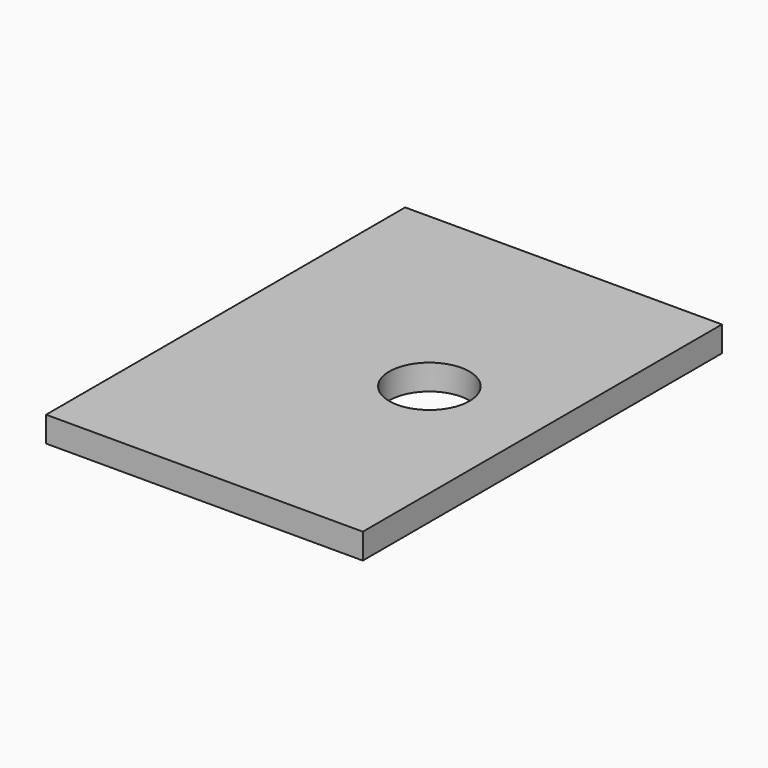
from build123d import *

# Parameters (mm, degrees)
F0_R     = 10
F1_DEPTH = 6.35
F2_W     = 124.221875
F2_H     = 111.91875
F2_R     = 10
F3_DEPTH = 6.351


# Not quite as in the source:
# - a feature names something its author has since deleted; it is built from what else it names


with BuildPart() as f1:
    # F0 (on Top) → F1 (new body)
    with BuildSketch(Plane.XY):
        Polygon((50.8, -55.959375), (50.8, 55.959375), (-50.8, 55.959375), (-152.4, 55.959375), (-152.4, -55.959375), (-50.8, -55.959375), align=None)
        with Locations((-101.6, 0)):
            Circle(F0_R, mode=Mode.SUBTRACT)
        Circle(F0_R, mode=Mode.SUBTRACT)
    extrude(amount=F1_DEPTH)

    # F2 (on face) → F3 (cut, through all)
    with BuildSketch(Plane.XY.offset(6.35)):
        with Locations((-11.3109375, 0)):
            Rectangle(F2_W, F2_H)
        Circle(F2_R, mode=Mode.SUBTRACT)
    extrude(amount=-F3_DEPTH, mode=Mode.SUBTRACT)


solid = f1.part
